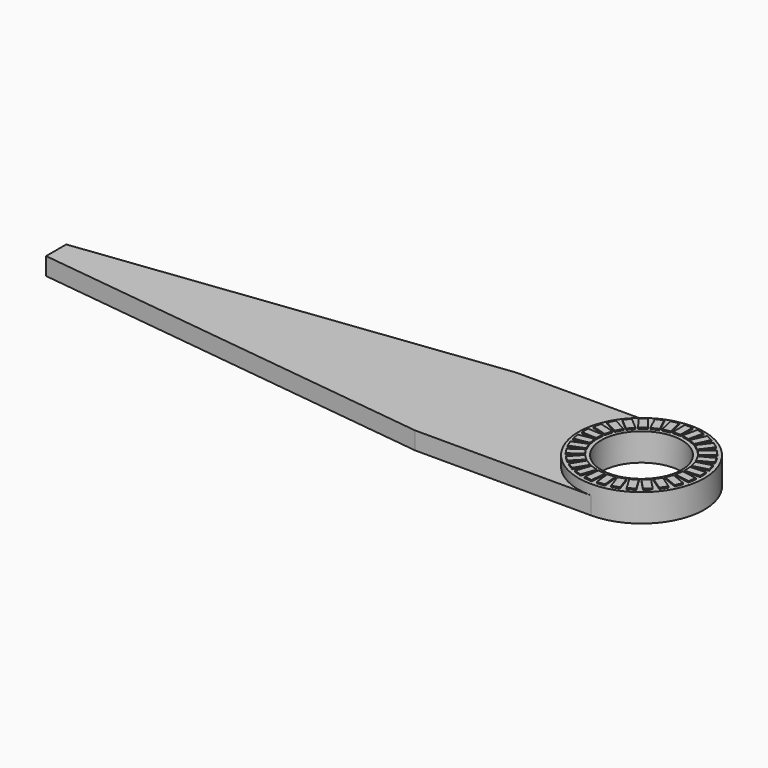
from build123d import *

# Parameters (mm, degrees)
F0_R         = 8
F1_DEPTH     = 3.5
F2_R         = 8
F3_DEPTH     = 2
F4_W         = 1.5
F4_H         = 3
F5_DEPTH     = 0.25
F6_TEXT_SIZE = 8.8383841406
F7_DEPTH     = 2
F8_W         = 20
F8_H         = 2
F9_DEPTH     = 2


# Not quite as in the source:
# - Text() gives the source's letters only with a copy of the font that has no kerning and outlines rounded to 1/6400 em; it was checked with that copy


with BuildPart() as f1:
    # F0 (on Top) → F1 (new body)
    with BuildSketch(Plane.XY):
        with BuildLine():
            ThreePointArc((0, -12.5), (-12.5, 0), (0, 12.5))
            Line((0, 12.5), (-35, 12.5))
            Line((-35, 12.5), (-116.3887844346, 2.5067138408))
            Line((-116.3887844346, 2.5067138408), (-116.3887844346, -2.5067138408))
            Line((-116.3887844346, -2.5067138408), (-35, -12.5))
            Line((-35, -12.5), (0, -12.5))
        make_face()
        with BuildLine():
            ThreePointArc((0, -12.5), (8.8388347648, -8.8388347648), (12.5, 0))
            ThreePointArc((12.5, 0), (8.8388347648, 8.8388347648), (0, 12.5))
            ThreePointArc((0, 12.5), (-12.5, 0), (0, -12.5))
        make_face()
        Circle(F0_R, mode=Mode.SUBTRACT)
    extrude(amount=F1_DEPTH)

    # F2 (on face) → F3 (join)
    with BuildSketch(Plane.XY.offset(3.5)):
        with BuildLine():
            ThreePointArc((0, -12.5), (8.8388347648, -8.8388347648), (12.5, 0))
            ThreePointArc((12.5, 0), (8.8388347648, 8.8388347648), (0, 12.5))
            ThreePointArc((0, 12.5), (-12.5, 0), (0, -12.5))
        make_face()
        Circle(F2_R, mode=Mode.SUBTRACT)
    extrude(amount=F3_DEPTH)

    # F4 (on face) → F5 (join)
    with BuildSketch(Plane.XY.offset(5.5)):
        with Locations((0, 10.25)):
            Rectangle(F4_W, F4_H)
        Polygon((2.6134567686, 8.3842020323), (3.2583680893, 11.3140636994), (1.7934372557, 11.6365193598), (1.1485259351, 8.7066576926), align=None)
        Polygon((4.3547112034, 7.626368096), (5.6143785081, 10.349094355), (4.2530153786, 10.9789280073), (2.9933480739, 8.2562017483), align=None)
        Polygon((5.8923441822, 6.5119336635), (7.7078668278, 8.9002128606), (6.5137272292, 9.8079741834), (4.6982045837, 7.4196949863), align=None)
        Polygon((7.154457696, 5.0930084505), (9.4409438613, 7.0351673048), (8.4698644342, 8.1784103875), (6.1833782688, 6.2362515332), align=None)
        Polygon((8.0820367194, 3.4359398228), (10.7325728528, 4.8411651449), (10.0299601917, 6.1664332116), (7.3794240584, 4.7612078895), align=None)
        Polygon((8.6317086884, 1.6182104677), (11.522358666, 2.4207954833), (11.1210661582, 3.8661204721), (8.2304161806, 3.0635354565), align=None)
        Polygon((8.7777715526, -0.2751846103), (11.7733717942, -0.1127678845), (11.6921634313, 1.3850322363), (8.6965631898, 1.2226155105), align=None)
        Polygon((8.5133955748, -2.1557123617), (11.4738751424, -2.6410583514), (11.7165481373, -1.1608185676), (8.7560685697, -0.6754725779), align=None)
        Polygon((7.8509426819, -3.9354413991), (10.6378728413, -5.0458558651), (11.1930800744, -3.6523907854), (8.4061499149, -2.5419763194), align=None)
        Polygon((6.8213884349, -5.5311535705), (9.3044554293, -7.2147147666), (10.1462360274, -5.9731812694), (7.6631690329, -4.2896200733), align=None)
        Polygon((5.472873646, -6.8682351485), (7.5359720226, -9.0462216242), (8.6249652605, -8.014672436), (6.5618668839, -5.8366859602), align=None)
        Polygon((3.8684533682, -7.8841656843), (5.4151149397, -10.4547372129), (6.700400704, -9.6814064271), (5.1537391324, -7.1108348986), align=None)
        Polygon((2.0831485103, -8.5314413955), (3.0410531007, -11.374400909), (4.4625328575, -10.8954486138), (3.5046282671, -8.0524891002), align=None)
        Polygon((0.2004379433, -8.7797963889), (0.5247949986, -11.7622102604), (2.0160019343, -11.6000317327), (1.6916448791, -8.6176178613), align=None)
        Polygon((-1.6916448791, -8.6176178613), (-2.0160019343, -11.6000317327), (-0.5247949986, -11.7622102604), (-0.2004379433, -8.7797963889), align=None)
        Polygon((-3.5046282671, -8.0524891002), (-4.4625328575, -10.8954486138), (-3.0410531007, -11.374400909), (-2.0831485103, -8.5314413955), align=None)
        Polygon((-5.1537391324, -7.1108348986), (-6.700400704, -9.6814064271), (-5.4151149397, -10.4547372129), (-3.8684533682, -7.8841656843), align=None)
        Polygon((-6.5618668839, -5.8366859602), (-8.6249652605, -8.014672436), (-7.5359720226, -9.0462216242), (-5.472873646, -6.8682351485), align=None)
        Polygon((-7.6631690329, -4.2896200733), (-10.1462360274, -5.9731812694), (-9.3044554293, -7.2147147666), (-6.8213884349, -5.5311535705), align=None)
        Polygon((-8.4061499149, -2.5419763194), (-11.1930800744, -3.6523907854), (-10.6378728413, -5.0458558651), (-7.8509426819, -3.9354413991), align=None)
        Polygon((-8.7560685697, -0.6754725779), (-11.7165481373, -1.1608185676), (-11.4738751424, -2.6410583514), (-8.5133955748, -2.1557123617), align=None)
        Polygon((-8.6965631898, 1.2226155105), (-11.6921634313, 1.3850322363), (-11.7733717942, -0.1127678845), (-8.7777715526, -0.2751846103), align=None)
        Polygon((-8.2304161806, 3.0635354565), (-11.1210661582, 3.8661204721), (-11.522358666, 2.4207954833), (-8.6317086884, 1.6182104677), align=None)
        Polygon((-7.3794240584, 4.7612078895), (-10.0299601917, 6.1664332116), (-10.7325728528, 4.8411651449), (-8.0820367194, 3.4359398228), align=None)
        Polygon((-6.1833782688, 6.2362515332), (-8.4698644342, 8.1784103875), (-9.4409438613, 7.0351673048), (-7.154457696, 5.0930084505), align=None)
        Polygon((-4.6982045837, 7.4196949863), (-6.5137272292, 9.8079741834), (-7.7078668278, 8.9002128606), (-5.8923441822, 6.5119336635), align=None)
        Polygon((-2.9933480739, 8.2562017483), (-4.2530153786, 10.9789280073), (-5.6143785081, 10.349094355), (-4.3547112034, 7.626368096), align=None)
        Polygon((-1.1485259351, 8.7066576926), (-1.7934372557, 11.6365193598), (-3.2583680893, 11.3140636994), (-2.6134567686, 8.3842020323), align=None)
    extrude(amount=F5_DEPTH)

    # F6 (on face) → F7 (cut)
    with BuildSketch(Plane(origin=(0, 0, 0), x_dir=(1, 0, 0), z_dir=(0, 0, -1))):
        with Locations((-67.0580267906, -3.0681819189)):
            Text('BMS ART', F6_TEXT_SIZE, font='Open Sans', font_style=FontStyle.ITALIC, text_align=(TextAlign.LEFT, TextAlign.BOTTOM))
    extrude(amount=-F7_DEPTH, mode=Mode.SUBTRACT)

    # F8 (on Top) → F9 (cut)
    with BuildSketch(Plane.XY):
        with Locations((-106.3887844346, 0.0067138408)):
            Rectangle(F8_W, F8_H)
    extrude(amount=F9_DEPTH, mode=Mode.SUBTRACT)


solid = f1.part
